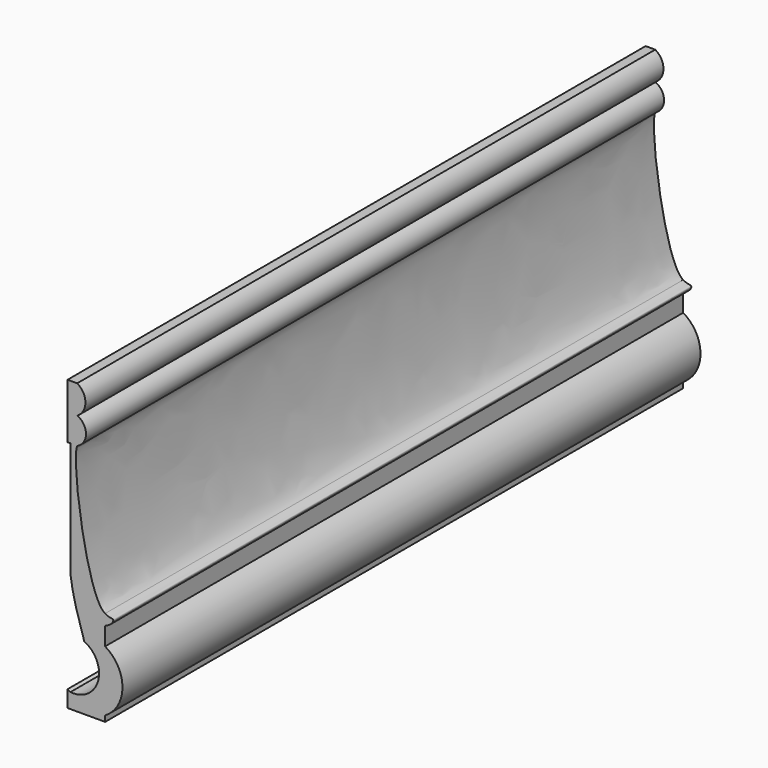
from build123d import *

# Parameters (mm, degrees)
F1_DEPTH = 25


with BuildPart() as f1:
    # F0 (on Front) → F1 (new body)
    with BuildSketch(Plane.XZ):
        with BuildLine():
            add(Edge.make_bspline(
                [(0, -2.5), (-0.0708144549, -2.4524918378), (-0.1956100643, -2.3687686762), (-0.3180885676, -2.1971845687), (-0.1116996866, -2.1227784123), (0, -2.0733320448)],
                knots=[0, 0, 0, 0, 0.0945574941, 0.1666377313, 0.2518567558, 0.2518567558, 0.2518567558, 0.2518567558], degree=3))
            Line((0, -2.5), (0, -2.0733320448))
        make_face()
        with BuildLine():
            Line((0, -2.7), (0, -2.5))
            add(Edge.make_bspline(
                [(0, -2.5), (-0.0708144549, -2.4524918378), (-0.1956100643, -2.3687686762), (-0.3180885676, -2.1971845687), (-0.1116996866, -2.1227784123), (0, -2.0733320448)],
                knots=[0, 0, 0, 0, 0.0945574941, 0.1666377313, 0.2518567558, 0.2518567558, 0.2518567558, 0.2518567558], degree=3))
            Line((0, -2.0733320448), (0, -1.6986069948))
            add(Edge.make_bspline(
                [(0, -1.6986069948), (-0.0383555824, -1.6741333918), (-0.6515753448, -1.1515664964), (-1.1755755053, 2.6788852088), (-0.9639657726, 3.0935284682), (-0.9623506631, 3.0964508274)],
                knots=[0.482349916, 0.482349916, 0.482349916, 0.482349916, 0.5109278826, 0.9233932624, 0.9264915283, 0.9264915283, 0.9264915283, 0.9264915283], degree=3))
            add(Edge.make_bspline(
                [(-0.9623506631, 3.0964508274), (-0.9410767081, 3.1349436593), (-0.9133074942, 3.1441076976), (-0.8826490073, 3.1402254678)],
                knots=[0.9264915283, 0.9264915283, 0.9264915283, 0.9264915283, 0.9673013749, 0.9673013749, 0.9673013749, 0.9673013749], degree=3))
            ThreePointArc((-0.8826490073, 3.1402254678), (-0.6635180881, 3.6029526705), (-0.9646388468, 4.0170313014))
            ThreePointArc((-0.9646388468, 4.0170313014), (-0.6816397602, 4.5092221063), (-0.9670821019, 5))
            Line((-0.9670821019, 5), (-1.3, 5))
            Line((-1.3, 5), (-1.3, 3.0956115703))
            Line((-1.3, 3.0956115703), (-1.2, 3.0958601291))
            Line((-1.2, 3.0958601291), (-1.2, 1.1517136591))
            Line((-1.2, 1.1517136591), (-1.2, -0.8931580232))
            add(Edge.make_bspline(
                [(-0.7223970163, -2.7801062833), (-0.921047879, -2.1601191709), (-1.119437918, -1.5398665045), (-1.2, -0.8931580232)],
                knots=[0.0003276246, 0.0003276246, 0.0003276246, 0.0003276246, 0.4939175623, 0.4939175623, 0.4939175623, 0.4939175623], degree=3))
            ThreePointArc((-0.7223970163, -2.7801062833), (-0.7217999511, -2.781163117), (-0.7208323102, -2.7818959578))
            ThreePointArc((-0.7208323102, -2.7818959578), (-0.2432721108, -3.8337162096), (-1.1993774544, -4.4819847944))
            ThreePointArc((-1.1993774544, -4.4819847944), (-1.199979754, -4.481857829), (-1.2005433473, -4.4816103465))
            Line((-1.2005433473, -4.4816103465), (-1.3, -4.4250912033))
            Line((-1.3, -4.4250912033), (-1.3, -5))
            Line((-1.3, -5), (0, -5))
            Line((0, -5), (0, -4.8))
            ThreePointArc((0, -4.8), (0.5995079207, -3.75), (0, -2.7))
        make_face()
        with BuildLine():
            Line((0, -1.6986069948), (0, -2.0733320448))
            add(Edge.make_bspline(
                [(0, -2.0733320448), (0.0594769695, -2.0470032325), (0.2344591808, -1.9618765045), (0.3482438258, -1.7339244568), (0.1300816825, -1.7816084057), (0, -1.6986069948)],
                knots=[0.2518567558, 0.2518567558, 0.2518567558, 0.2518567558, 0.2972335109, 0.3854286924, 0.482349916, 0.482349916, 0.482349916, 0.482349916], degree=3))
        make_face()
        with BuildLine():
            add(Edge.make_bspline(
                [(-0.9623506631, 3.0964508274), (-0.9410767081, 3.1349436593), (-0.9133074942, 3.1441076976), (-0.8826490073, 3.1402254678)],
                knots=[0.9264915283, 0.9264915283, 0.9264915283, 0.9264915283, 0.9673013749, 0.9673013749, 0.9673013749, 0.9673013749], degree=3))
            ThreePointArc((-0.9623506631, 3.0964508274), (-0.9215059833, 3.1165286149), (-0.8826490073, 3.1402254678))
        make_face()
    extrude(amount=F1_DEPTH)


solid = f1.part
